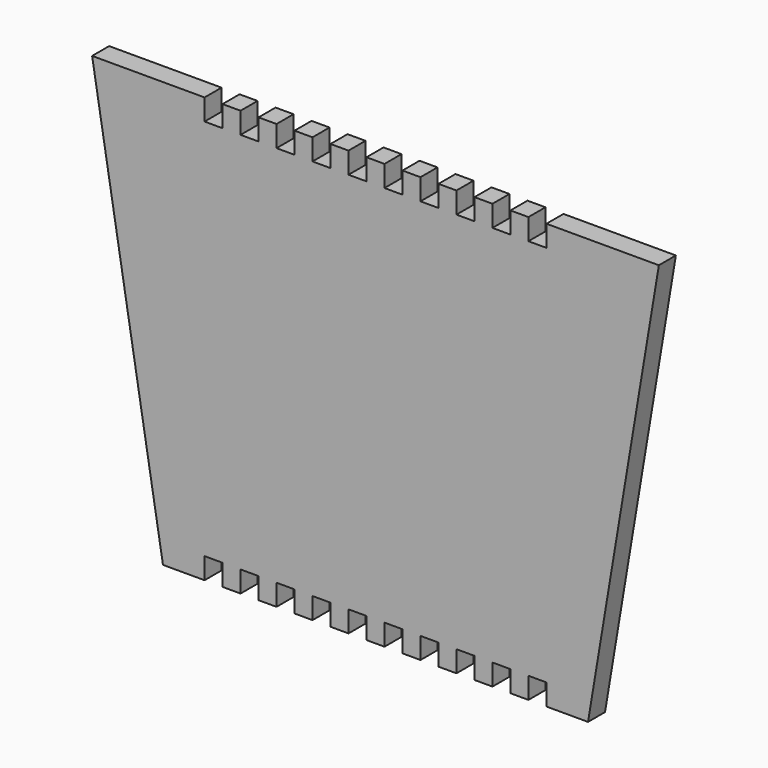
from build123d import *

# Parameters (mm, degrees)
F1_DEPTH = 15


# Not quite as in the source:
# - a feature names something its author has since deleted; it is built from what else it names


with BuildPart() as f1:
    # F0 (on Front) → F1 (new body)
    with BuildSketch(Plane.XZ):
        Polygon((150, -150), (200, 150), (120.65, 150), (120.65, 135), (107.95, 135), (107.95, 150), (95.25, 150), (95.25, 135), (82.55, 135), (82.55, 150), (69.85, 150), (69.85, 135), (57.15, 135), (57.15, 150), (44.45, 150), (44.45, 135), (31.75, 135), (31.75, 150), (19.05, 150), (19.05, 135), (6.35, 135), (6.35, 150), (0, 150), (-6.35, 150), (-6.35, 135), (-19.05, 135), (-19.05, 150), (-31.75, 150), (-31.75, 135), (-44.45, 135), (-44.45, 150), (-57.15, 150), (-57.15, 135), (-69.85, 135), (-69.85, 150), (-82.55, 150), (-82.55, 135), (-95.25, 135), (-95.25, 150), (-107.95, 150), (-107.95, 135), (-120.65, 135), (-120.65, 150), (-200, 150), (-150, -150), (-120.65, -150), (-120.65, -135), (-107.95, -135), (-107.95, -150), (-95.25, -150), (-95.25, -135), (-82.55, -135), (-82.55, -150), (-69.85, -150), (-69.85, -135), (-57.15, -135), (-57.15, -150), (-44.45, -150), (-44.45, -135), (-31.75, -135), (-31.75, -150), (-19.05, -150), (-19.05, -135), (-6.35, -135), (-6.35, -150), (0, -150), (6.35, -150), (6.35, -135), (19.05, -135), (19.05, -150), (31.75, -150), (31.75, -135), (44.45, -135), (44.45, -150), (57.15, -150), (57.15, -135), (69.85, -135), (69.85, -150), (82.55, -150), (82.55, -135), (95.25, -135), (95.25, -150), (107.95, -150), (107.95, -135), (120.65, -135), (120.65, -150), align=None)
    extrude(amount=F1_DEPTH)


solid = f1.part
